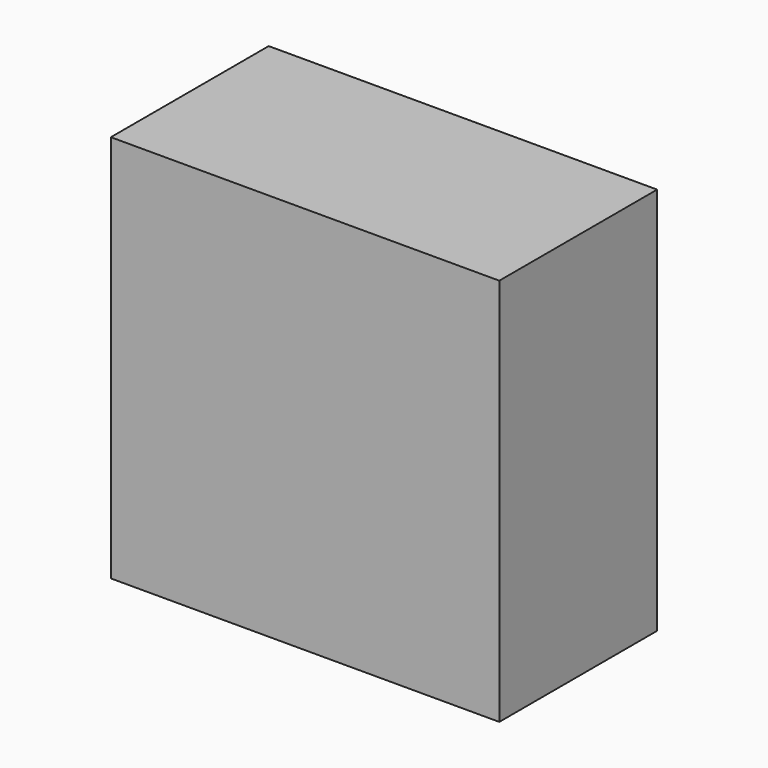
from build123d import *

# Parameters (mm, degrees)
F1_W     = 8.001
F1_H     = 8.001
F2_DEPTH = 4.064


# Not quite as in the source:
# - a variable given as a bare number and used for a length is read in inches; the dataset says mm whatever the document's units were


with BuildPart() as f2:
    # F1 (on Front) → F2 (new body)
    with BuildSketch(Plane.XZ):
        Rectangle(F1_W, F1_H)
    extrude(amount=F2_DEPTH)


solid = f2.part
